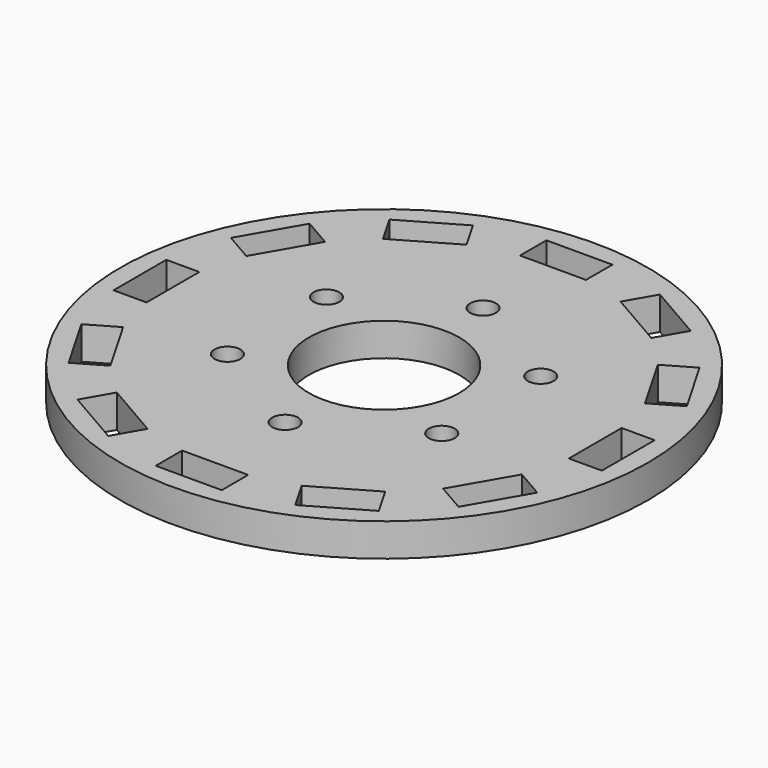
from build123d import *

# Parameters (mm, degrees)
F0_R            = 50.8
F0_R_2          = 14.478
F1_DEPTH        = 6.35
F2_R            = 2.4892
F3_DEPTH        = 25.4
F3_COPIES_COUNT = 6
F4_W            = 12.7
F4_H            = 6.35
F5_DEPTH        = 25.4
F5_COPIES_COUNT = 12


# Not quite as in the source:
# - a pattern or mirror of a feature is missing from the dataset's text; its kind, count and spacing are read off the source's solid


with BuildPart() as f1:
    # F0 (on Top) → F1 (new body)
    with BuildSketch(Plane.XY):
        Circle(F0_R)
        Circle(F0_R_2, mode=Mode.SUBTRACT)
    extrude(amount=F1_DEPTH)

    # F2 (on face) → F3 (cut)
    with BuildSketch(Plane.XY.offset(6.35)):
        with Locations((0, 23.8125)):
            Circle(F2_R)
    f3 = extrude(amount=-F3_DEPTH, mode=Mode.SUBTRACT)

    # F3_copies: F3 ×6 about axis
    f3_copies_axis = Axis((0, 0, 0), (0, 0, 1))
    for i in range(1, F3_COPIES_COUNT):
        add(f3.rotate(f3_copies_axis, i * 360 / F3_COPIES_COUNT), mode=Mode.SUBTRACT)

    # F4 (on face) → F5 (cut)
    with BuildSketch(Plane.XY.offset(6.35)):
        with Locations((0, 43.815)):
            Rectangle(F4_W, F4_H)
    f5 = extrude(amount=-F5_DEPTH, mode=Mode.SUBTRACT)

    # F5_copies: F5 ×12 about axis
    f5_copies_axis = Axis((0, 0, 0), (0, 0, 1))
    for i in range(1, F5_COPIES_COUNT):
        add(f5.rotate(f5_copies_axis, i * 360 / F5_COPIES_COUNT), mode=Mode.SUBTRACT)


solid = f1.part
